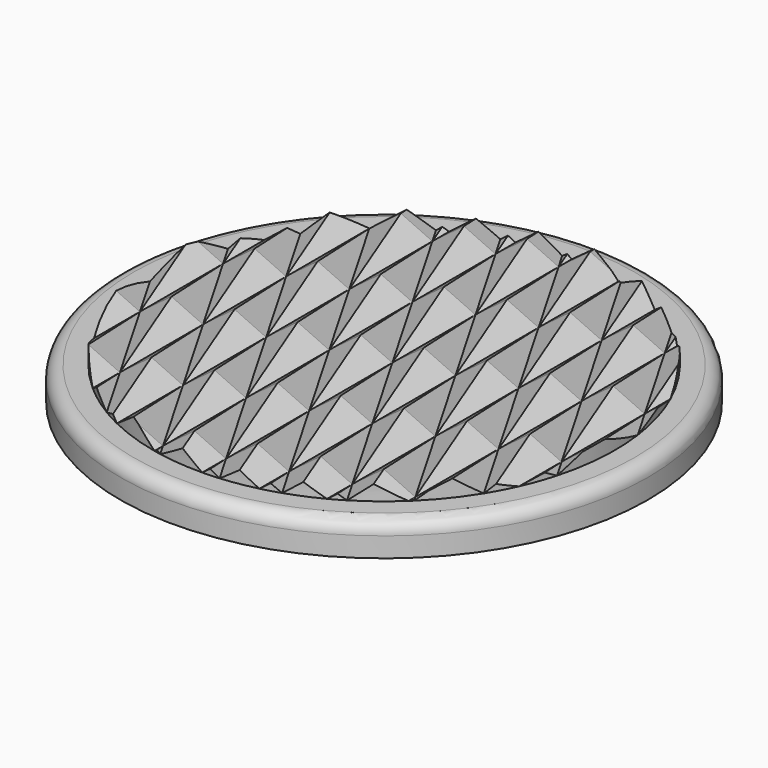
from build123d import *

# Parameters (mm, degrees)
F0_R     = 50.8
F0_R_2   = 44.45
F1_DEPTH = 6.35
F2_DEPTH = 10
F7_DEPTH = 88.9
F9_DEPTH = 88.9


# Not quite as in the source:
# - a fillet or chamfer that OpenCascade refuses, or shapes differently, is made with other operations: its cross-section is extruded or revolved along the edge and cut away or added


with BuildPart() as f1:
    # F0 (on Top) → F1 (new body)
    with BuildSketch(Plane.XY):
        Circle(F0_R)
        Circle(F0_R_2, mode=Mode.SUBTRACT)
    extrude(amount=F1_DEPTH)

    # F0 (on Top) → F2 (join)
    with BuildSketch(Plane.XY):
        Circle(F0_R_2)
    extrude(amount=F2_DEPTH)

    # F6 (on face) → F7 (cut)
    with BuildSketch(Plane(origin=(0, -44.45, 0), x_dir=(-1, 0, 0), z_dir=(0, 1, 0))):
        Polygon((39.45, 6.35), (44.45, 10), (34.45, 10), align=None)
        Polygon((29.45, 6.35), (34.45, 10), (24.45, 10), align=None)
        Polygon((19.4500000001, 6.35), (24.45, 10), (14.4500000001, 10), align=None)
        Polygon((9.4500000001, 6.35), (14.4500000001, 10), (4.4500000002, 10), align=None)
        Polygon((-0.5499999998, 6.35), (4.4500000002, 10), (-5.5499999998, 10), align=None)
        Polygon((-10.5499999998, 6.35), (-5.5499999998, 10), (-15.5499999998, 10), align=None)
        Polygon((-20.5499999997, 6.35), (-15.5499999998, 10), (-25.5499999997, 10), align=None)
        Polygon((-30.5499999997, 6.35), (-25.5499999997, 10), (-35.5499999997, 10), align=None)
        Polygon((-40.5499999997, 6.35), (-35.5499999997, 10), (-45.5499999996, 10), align=None)
    extrude(amount=F7_DEPTH, mode=Mode.SUBTRACT)

    # F8 (on face) → F9 (cut)
    with BuildSketch(Plane(origin=(22.225, -38.4948291982, 0), x_dir=(0.8660254038, 0.5, 0), z_dir=(0.5, -0.8660254038, 0))):
        Polygon((-33.8791470656, 10), (-43.8791470656, 10), (-38.8791470656, 6.35), align=None)
        Polygon((-23.8791470657, 10), (-33.8791470656, 10), (-28.8791470656, 6.35), align=None)
        Polygon((-13.8791470657, 10), (-23.8791470657, 10), (-18.8791470657, 6.35), align=None)
        Polygon((-3.8791470657, 10), (-13.8791470657, 10), (-8.8791470657, 6.35), align=None)
        Polygon((6.1208529342, 10), (-3.8791470657, 10), (1.1208529342, 6.35), align=None)
        Polygon((16.1208529342, 10), (6.1208529342, 10), (11.1208529342, 6.35), align=None)
        Polygon((26.1208529341, 10), (16.1208529342, 10), (21.1208529342, 6.35), align=None)
        Polygon((36.1208529341, 10), (26.1208529341, 10), (31.1208529341, 6.35), align=None)
        Polygon((46.1208529341, 10), (36.1208529341, 10), (41.1208529341, 6.35), align=None)
    extrude(amount=-F9_DEPTH, mode=Mode.SUBTRACT)

    # F10: fillet of radius 2.54 on 1 edges, made by hand

    # F10_s1 → F10_t2 (revolve, cut)
    with BuildSketch(Plane.XZ):
        with BuildLine():
            ThreePointArc((50.8, 3.81), (50.0560512242, 5.6060512242), (48.26, 6.35))
            Line((48.26, 6.35), (50.8, 6.35))
            Line((50.8, 6.35), (50.8, 3.81))
        make_face()
    revolve(axis=Axis((0, 0, 6.35), (0, 0, -1)), mode=Mode.SUBTRACT)


solid = f1.part
